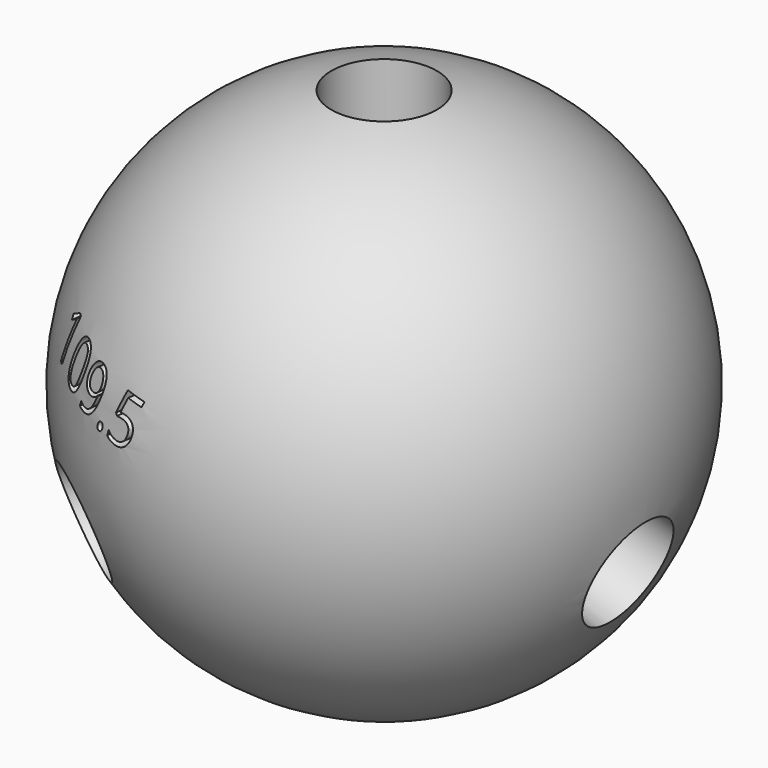
from build123d import *

# Parameters (mm, degrees)
F6_R          = 3.175
F7_DEPTH      = 38.1
F8_ANGLE      = 109.5
F9_ANGLE      = 109.5
F10_ANGLE     = 125
F12_TEXT_SIZE = 3.3307251417
F13_DEPTH     = 10.16


# Not quite as in the source:
# - Text() gives the source's letters only with a copy of the font that has no kerning and outlines rounded to 1/6400 em; it was checked with that copy


with BuildPart() as f2:
    # F0 (on Front) → F2 (revolve)
    with BuildSketch(Plane.XZ):
        with BuildLine():
            Line((0, -15.875), (0, 15.875))
            ThreePointArc((0, 15.875), (-15.875, 0), (0, -15.875))
        make_face()
    revolve(axis=Axis((0, 0, 0), (0, 0, 1)))

    # F12 (on offset) → F13 (cut)
    with BuildSketch(Plane(origin=(-10.427869036, -14.6193332101, -6.3590206684), x_dir=(0.8368745679, -0.5019642676, -0.2183410903), z_dir=(-0.5473947001, -0.7674190661, -0.3338068592))):
        with Locations((-3.5207134206, 7.6729832217)):
            Text('109.5', F12_TEXT_SIZE, font='Open Sans', text_align=(TextAlign.LEFT, TextAlign.BOTTOM))
    extrude(amount=-F13_DEPTH, mode=Mode.SUBTRACT)


with BuildPart() as f7:
    # F6 (on offset) → F7 (new body)
    with BuildSketch(Plane.XY.offset(6.35)):
        Circle(F6_R)
    extrude(amount=F7_DEPTH)


with BuildPart() as f8_1:
    # F8: copy of F7
    add(f7.part.rotate(Axis((0, 36.7893390357, 0), (0, 1, 0)), F8_ANGLE))


with BuildPart() as f9_1:
    # F9: copy of F8_1
    add(f8_1.part.rotate(Axis((0, 0, 33.9551977813), (0, 0, 1)), F9_ANGLE))


with BuildPart() as f10_1:
    # F10: copy of F9_1
    add(f9_1.part.rotate(Axis((0, 0, 44.45), (0, 0, 1)), F10_ANGLE))


with BuildPart() as f2_1:
    add(f2.part)

    # F14: cut F7, F10_1, F9_1, F8_1
    add(f7.part, mode=Mode.SUBTRACT)
    add(f10_1.part, mode=Mode.SUBTRACT)
    add(f9_1.part, mode=Mode.SUBTRACT)
    add(f8_1.part, mode=Mode.SUBTRACT)


solid = f2_1.part
